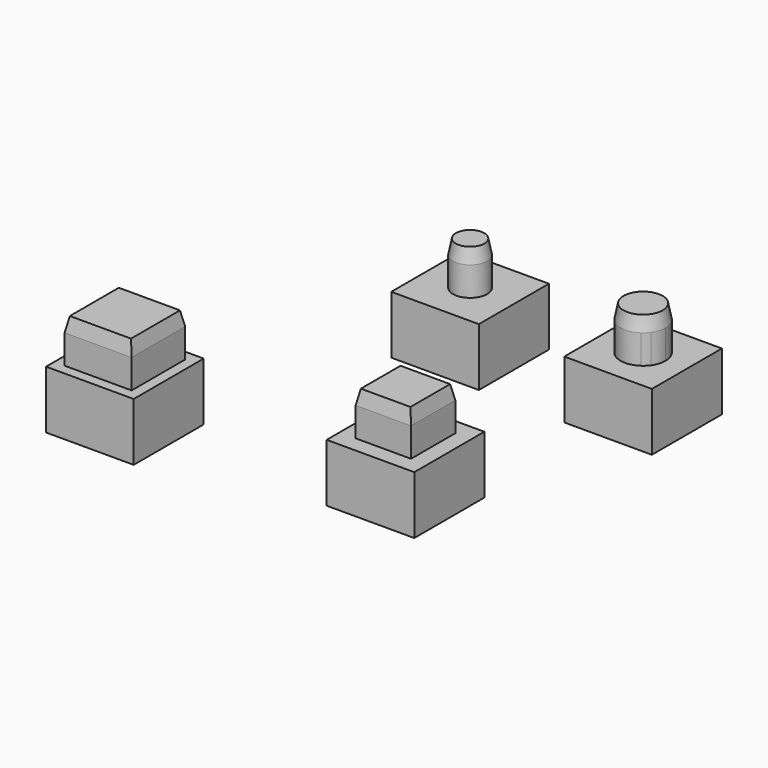
from build123d import *

# Parameters (mm, degrees)
F0_W          = 7.6708
F0_H          = 7.6708
F0_W_2        = 5.8674
F0_H_2        = 5.8674
F0_W_3        = 3.2258
F0_H_3        = 3.2258
F1_DEPTH      = 5.08
F0_R          = 1.4986
F0_W_4        = 4.8514
F0_H_4        = 4.8514
F2_DEPTH      = 8.89
F3_DEPTH      = 8.89
F4_DEPTH      = 8.89
F5_DEPTH      = 8.89
F6_C1_SIZE2   = 0.254
F6_C1_SIZE    = 1.27
F6_C2_SIZE2   = 0.254
F6_C2_SIZE    = 1.27
F6_C3_SIZE2   = 0.254
F6_C3_SIZE    = 1.27
F6_C4_SIZE2   = 0.254
F6_C4_SIZE    = 1.27
F6_4_C1_SIZE2 = 0.254
F6_4_C1_SIZE  = 1.27
F6_4_C2_SIZE2 = 0.254
F6_4_C2_SIZE  = 1.27
F6_4_C3_SIZE2 = 0.254
F6_4_C3_SIZE  = 1.27
F6_4_C4_SIZE2 = 0.254
F6_4_C4_SIZE  = 1.27
F7_DEPTH      = 3.302
F8_DEPTH      = 3.302
F9_DEPTH      = 3.302
F10_DEPTH     = 3.302


# Not quite as in the source:
# - a fillet or chamfer that OpenCascade refuses, or shapes differently, is made with other operations: its cross-section is extruded or revolved along the edge and cut away or added


with BuildPart() as f1:
    # F0 (on Top) → F1 (new body)
    with BuildSketch(Plane.XY):
        with Locations((3.9261005717, 4.6390335905)):
            Rectangle(F0_W, F0_H)
        with Locations((3.9261005717, 4.6390335905)):
            Rectangle(F0_W_2, F0_H_2, mode=Mode.SUBTRACT)
        with Locations((3.9261005717, 4.6390335905)):
            Rectangle(F0_W_2, F0_H_2)
        with Locations((3.9261005717, 4.6390335905)):
            Rectangle(F0_W_3, F0_H_3, mode=Mode.SUBTRACT)
        with Locations((3.9261005717, 4.6390335905)):
            Rectangle(F0_W_3, F0_H_3)
    extrude(amount=F1_DEPTH)

    # F0 (on Top) → F5 (join)
    with BuildSketch(Plane.XY):
        with Locations((3.9261005717, 4.6390335905)):
            Rectangle(F0_W_2, F0_H_2)
        with Locations((3.9261005717, 4.6390335905)):
            Rectangle(F0_W_3, F0_H_3, mode=Mode.SUBTRACT)
        with Locations((3.9261005717, 4.6390335905)):
            Rectangle(F0_W_3, F0_H_3)
    extrude(amount=F5_DEPTH)

    # F6: chamfer of 0.254 x 1.27 on 4 edges, made by hand

    # F6_c1
    f6_c1_edges = [f1.edges().sort_by_distance(p)[0] for p in [
        (3.9261005717, 1.7053335905, 8.89),
    ]]
    f6_c1_side = f1.faces().sort_by_distance((3.9261005717, 1.7053335905, 8.88492))[0]
    chamfer(f6_c1_edges, length=F6_C1_SIZE, length2=F6_C1_SIZE2, reference=f6_c1_side)

    # F6_c2
    f6_c2_edges = [f1.edges().sort_by_distance(p)[0] for p in [
        (6.8598005717, 4.7660335905, 8.89),
    ]]
    f6_c2_side = f1.faces().sort_by_distance((6.8598005717, 4.7660335905, 8.88492))[0]
    chamfer(f6_c2_edges, length=F6_C2_SIZE, length2=F6_C2_SIZE2, reference=f6_c2_side)

    # F6_c3
    f6_c3_edges = [f1.edges().sort_by_distance(p)[0] for p in [
        (3.7991005717, 7.5727335905, 8.89),
    ]]
    f6_c3_side = f1.faces().sort_by_distance((3.7991005717, 7.5727335905, 8.88492))[0]
    chamfer(f6_c3_edges, length=F6_C3_SIZE, length2=F6_C3_SIZE2, reference=f6_c3_side)

    # F6_c4
    f6_c4_edges = [f1.edges().sort_by_distance(p)[0] for p in [
        (0.9924005717, 4.6390335905, 8.89),
    ]]
    f6_c4_side = f1.faces().sort_by_distance((0.9924005717, 4.6390335905, 8.88492))[0]
    chamfer(f6_c4_edges, length=F6_C4_SIZE, length2=F6_C4_SIZE2, reference=f6_c4_side)

    # F0 (on Top) → F10 (cut)
    with BuildSketch(Plane.XY):
        with Locations((3.9261005717, 4.6390335905)):
            Rectangle(F0_W_3, F0_H_3)
    extrude(amount=F10_DEPTH, mode=Mode.SUBTRACT)


with BuildPart() as f1b:
    # F0 (on Top) → F1, piece 2 (new body)
    with BuildSketch(Plane.XY):
        with Locations((30.6640900671, 27.9408358037)):
            Rectangle(F0_W, F0_H)
        with BuildLine():
            Line((29.0511900671, 29.0693506862), (29.0511900671, 29.5537358037))
            Line((29.0511900671, 29.5537358037), (29.5355751847, 29.5537358037))
            ThreePointArc((29.5355751847, 29.5537358037), (30.6640900671, 29.9093358037), (31.7926049496, 29.5537358037))
            Line((31.7926049496, 29.5537358037), (32.2769900671, 29.5537358037))
            Line((32.2769900671, 29.5537358037), (32.2769900671, 29.0693506862))
            ThreePointArc((32.2769900671, 29.0693506862), (32.5415865252, 28.5324431904), (32.6325900671, 27.9408358037))
            ThreePointArc((32.6325900671, 27.9408358037), (32.5415865252, 27.349228417), (32.2769900671, 26.8123209213))
            Line((32.2769900671, 26.8123209213), (32.2769900671, 26.3279358037))
            Line((32.2769900671, 26.3279358037), (31.7926049496, 26.3279358037))
            ThreePointArc((31.7926049496, 26.3279358037), (30.6640900671, 25.9723358037), (29.5355751847, 26.3279358037))
            Line((29.5355751847, 26.3279358037), (29.0511900671, 26.3279358037))
            Line((29.0511900671, 26.3279358037), (29.0511900671, 26.8123209213))
            ThreePointArc((29.0511900671, 26.8123209213), (28.6955900671, 27.9408358037), (29.0511900671, 29.0693506862))
        make_face(mode=Mode.SUBTRACT)
        with BuildLine():
            Line((31.7926049496, 29.5537358037), (29.5355751847, 29.5537358037))
            ThreePointArc((29.5355751847, 29.5537358037), (29.2721503684, 29.3327755025), (29.0511900671, 29.0693506862))
            Line((29.0511900671, 29.0693506862), (29.0511900671, 26.8123209213))
            ThreePointArc((29.0511900671, 26.8123209213), (29.2721503684, 26.548896105), (29.5355751847, 26.3279358037))
            Line((29.5355751847, 26.3279358037), (31.7926049496, 26.3279358037))
            ThreePointArc((31.7926049496, 26.3279358037), (32.0560297659, 26.548896105), (32.2769900671, 26.8123209213))
            Line((32.2769900671, 26.8123209213), (32.2769900671, 29.0693506862))
            ThreePointArc((32.2769900671, 29.0693506862), (32.0560297659, 29.3327755025), (31.7926049496, 29.5537358037))
        make_face()
        with BuildLine():
            Line((29.0511900671, 26.8123209213), (29.0511900671, 29.0693506862))
            ThreePointArc((29.0511900671, 29.0693506862), (28.6955900671, 27.9408358037), (29.0511900671, 26.8123209213))
        make_face()
        with BuildLine():
            ThreePointArc((32.6325900671, 27.9408358037), (32.5415865252, 28.5324431904), (32.2769900671, 29.0693506862))
            Line((32.2769900671, 29.0693506862), (32.2769900671, 26.8123209213))
            ThreePointArc((32.2769900671, 26.8123209213), (32.5415865252, 27.349228417), (32.6325900671, 27.9408358037))
        make_face()
        with BuildLine():
            Line((31.7926049496, 26.3279358037), (29.5355751847, 26.3279358037))
            ThreePointArc((29.5355751847, 26.3279358037), (30.6640900671, 25.9723358037), (31.7926049496, 26.3279358037))
        make_face()
        with BuildLine():
            ThreePointArc((31.7926049496, 29.5537358037), (30.6640900671, 29.9093358037), (29.5355751847, 29.5537358037))
            Line((29.5355751847, 29.5537358037), (31.7926049496, 29.5537358037))
        make_face()
        with BuildLine():
            ThreePointArc((29.5355751847, 26.3279358037), (29.2721503684, 26.548896105), (29.0511900671, 26.8123209213))
            Line((29.0511900671, 26.8123209213), (29.0511900671, 26.3279358037))
            Line((29.0511900671, 26.3279358037), (29.5355751847, 26.3279358037))
        make_face()
        with BuildLine():
            Line((29.5355751847, 29.5537358037), (29.0511900671, 29.5537358037))
            Line((29.0511900671, 29.5537358037), (29.0511900671, 29.0693506862))
            ThreePointArc((29.0511900671, 29.0693506862), (29.2721503684, 29.3327755025), (29.5355751847, 29.5537358037))
        make_face()
        with BuildLine():
            Line((32.2769900671, 29.5537358037), (31.7926049496, 29.5537358037))
            ThreePointArc((31.7926049496, 29.5537358037), (32.0560297659, 29.3327755025), (32.2769900671, 29.0693506862))
            Line((32.2769900671, 29.0693506862), (32.2769900671, 29.5537358037))
        make_face()
        with BuildLine():
            Line((32.2769900671, 26.3279358037), (32.2769900671, 26.8123209213))
            ThreePointArc((32.2769900671, 26.8123209213), (32.0560297659, 26.548896105), (31.7926049496, 26.3279358037))
            Line((31.7926049496, 26.3279358037), (32.2769900671, 26.3279358037))
        make_face()
    extrude(amount=F1_DEPTH)

    # F0 (on Top) → F2 (join)
    with BuildSketch(Plane.XY):
        with BuildLine():
            Line((31.7926049496, 26.3279358037), (29.5355751847, 26.3279358037))
            ThreePointArc((29.5355751847, 26.3279358037), (30.6640900671, 25.9723358037), (31.7926049496, 26.3279358037))
        make_face()
        with BuildLine():
            Line((31.7926049496, 29.5537358037), (29.5355751847, 29.5537358037))
            ThreePointArc((29.5355751847, 29.5537358037), (29.2721503684, 29.3327755025), (29.0511900671, 29.0693506862))
            Line((29.0511900671, 29.0693506862), (29.0511900671, 26.8123209213))
            ThreePointArc((29.0511900671, 26.8123209213), (29.2721503684, 26.548896105), (29.5355751847, 26.3279358037))
            Line((29.5355751847, 26.3279358037), (31.7926049496, 26.3279358037))
            ThreePointArc((31.7926049496, 26.3279358037), (32.0560297659, 26.548896105), (32.2769900671, 26.8123209213))
            Line((32.2769900671, 26.8123209213), (32.2769900671, 29.0693506862))
            ThreePointArc((32.2769900671, 29.0693506862), (32.0560297659, 29.3327755025), (31.7926049496, 29.5537358037))
        make_face()
        with BuildLine():
            Line((29.0511900671, 26.8123209213), (29.0511900671, 29.0693506862))
            ThreePointArc((29.0511900671, 29.0693506862), (28.6955900671, 27.9408358037), (29.0511900671, 26.8123209213))
        make_face()
        with BuildLine():
            ThreePointArc((31.7926049496, 29.5537358037), (30.6640900671, 29.9093358037), (29.5355751847, 29.5537358037))
            Line((29.5355751847, 29.5537358037), (31.7926049496, 29.5537358037))
        make_face()
        with BuildLine():
            ThreePointArc((32.6325900671, 27.9408358037), (32.5415865252, 28.5324431904), (32.2769900671, 29.0693506862))
            Line((32.2769900671, 29.0693506862), (32.2769900671, 26.8123209213))
            ThreePointArc((32.2769900671, 26.8123209213), (32.5415865252, 27.349228417), (32.6325900671, 27.9408358037))
        make_face()
    extrude(amount=F2_DEPTH)

    # F6#2: chamfer of 0.254 x 1.27 on 1 edges, made by hand

    # F6_2_s1 → F6_2_t2 (revolve, cut)
    with BuildSketch(Plane(origin=(23.202503455, 33.1615633992, 0), x_dir=(0, 0, 1), z_dir=(-0.5732867069, -0.8193548387, 0))):
        Polygon((7.62, -11.0751608258), (8.89, -10.8211608258), (8.89, -11.0751608258), align=None)
    revolve(axis=Axis((30.6640900671, 27.9408358037, 8.89), (0, 0, 1)), mode=Mode.SUBTRACT)

    # F0 (on Top) → F7 (cut)
    with BuildSketch(Plane.XY):
        with BuildLine():
            Line((31.7926049496, 29.5537358037), (29.5355751847, 29.5537358037))
            ThreePointArc((29.5355751847, 29.5537358037), (29.2721503684, 29.3327755025), (29.0511900671, 29.0693506862))
            Line((29.0511900671, 29.0693506862), (29.0511900671, 26.8123209213))
            ThreePointArc((29.0511900671, 26.8123209213), (29.2721503684, 26.548896105), (29.5355751847, 26.3279358037))
            Line((29.5355751847, 26.3279358037), (31.7926049496, 26.3279358037))
            ThreePointArc((31.7926049496, 26.3279358037), (32.0560297659, 26.548896105), (32.2769900671, 26.8123209213))
            Line((32.2769900671, 26.8123209213), (32.2769900671, 29.0693506862))
            ThreePointArc((32.2769900671, 29.0693506862), (32.0560297659, 29.3327755025), (31.7926049496, 29.5537358037))
        make_face()
        with BuildLine():
            ThreePointArc((29.5355751847, 26.3279358037), (29.2721503684, 26.548896105), (29.0511900671, 26.8123209213))
            Line((29.0511900671, 26.8123209213), (29.0511900671, 26.3279358037))
            Line((29.0511900671, 26.3279358037), (29.5355751847, 26.3279358037))
        make_face()
        with BuildLine():
            Line((32.2769900671, 26.3279358037), (32.2769900671, 26.8123209213))
            ThreePointArc((32.2769900671, 26.8123209213), (32.0560297659, 26.548896105), (31.7926049496, 26.3279358037))
            Line((31.7926049496, 26.3279358037), (32.2769900671, 26.3279358037))
        make_face()
        with BuildLine():
            Line((32.2769900671, 29.5537358037), (31.7926049496, 29.5537358037))
            ThreePointArc((31.7926049496, 29.5537358037), (32.0560297659, 29.3327755025), (32.2769900671, 29.0693506862))
            Line((32.2769900671, 29.0693506862), (32.2769900671, 29.5537358037))
        make_face()
        with BuildLine():
            Line((29.5355751847, 29.5537358037), (29.0511900671, 29.5537358037))
            Line((29.0511900671, 29.5537358037), (29.0511900671, 29.0693506862))
            ThreePointArc((29.0511900671, 29.0693506862), (29.2721503684, 29.3327755025), (29.5355751847, 29.5537358037))
        make_face()
    extrude(amount=F7_DEPTH, mode=Mode.SUBTRACT)


with BuildPart() as f1c:
    # F0 (on Top) → F1, piece 3 (new body)
    with BuildSketch(Plane.XY):
        with Locations((15.4350250959, 28.039496392)):
            Rectangle(F0_W, F0_H)
        with Locations((15.4350250959, 28.039496392)):
            Rectangle(F0_W_3, F0_H_3, mode=Mode.SUBTRACT)
        with Locations((15.4350250959, 28.039496392)):
            Rectangle(F0_W_3, F0_H_3)
        with Locations((15.4350250959, 28.039496392)):
            Circle(F0_R, mode=Mode.SUBTRACT)
        with Locations((15.4350250959, 28.039496392)):
            Circle(F0_R)
    extrude(amount=F1_DEPTH)

    # F0 (on Top) → F3 (join)
    with BuildSketch(Plane.XY):
        with Locations((15.4350250959, 28.039496392)):
            Circle(F0_R)
    extrude(amount=F3_DEPTH)

    # F6#3: chamfer of 0.254 x 1.27 on 1 edges, made by hand

    # F6_3_s1 → F6_3_t2 (revolve, cut)
    with BuildSketch(Plane.XZ.offset(-28.039496392)):
        Polygon((16.9336250959, 7.62), (16.6796250959, 8.89), (16.9336250959, 8.89), align=None)
    revolve(axis=Axis((15.4350250959, 28.039496392, 8.89), (0, 0, 1)), mode=Mode.SUBTRACT)

    # F0 (on Top) → F8 (cut)
    with BuildSketch(Plane.XY):
        with Locations((15.4350250959, 28.039496392)):
            Rectangle(F0_W_3, F0_H_3)
        with Locations((15.4350250959, 28.039496392)):
            Circle(F0_R, mode=Mode.SUBTRACT)
        with Locations((15.4350250959, 28.039496392)):
            Circle(F0_R)
    extrude(amount=F8_DEPTH, mode=Mode.SUBTRACT)


with BuildPart() as f1d:
    # F0 (on Top) → F1, piece 4 (new body)
    with BuildSketch(Plane.XY):
        with Locations((25.6800069869, 8.162417023)):
            Rectangle(F0_W, F0_H)
        with Locations((25.6800069869, 8.162417023)):
            Rectangle(F0_W_4, F0_H_4, mode=Mode.SUBTRACT)
        with Locations((25.6800069869, 8.162417023)):
            Rectangle(F0_W_4, F0_H_4)
        with Locations((25.6800069869, 8.162417023)):
            Rectangle(F0_W_3, F0_H_3, mode=Mode.SUBTRACT)
        with Locations((25.6800069869, 8.162417023)):
            Rectangle(F0_W_3, F0_H_3)
    extrude(amount=F1_DEPTH)

    # F0 (on Top) → F4 (join)
    with BuildSketch(Plane.XY):
        with Locations((25.6800069869, 8.162417023)):
            Rectangle(F0_W_4, F0_H_4)
        with Locations((25.6800069869, 8.162417023)):
            Rectangle(F0_W_3, F0_H_3, mode=Mode.SUBTRACT)
        with Locations((25.6800069869, 8.162417023)):
            Rectangle(F0_W_3, F0_H_3)
    extrude(amount=F4_DEPTH)

    # F6#4: chamfer of 0.254 x 1.27 on 4 edges, made by hand

    # F6_4_c1
    f6_4_c1_edges = [f1d.edges().sort_by_distance(p)[0] for p in [
        (25.6800069869, 10.588117023, 8.89),
    ]]
    f6_4_c1_side = f1d.faces().sort_by_distance((25.6800069869, 10.588117023, 8.88492))[0]
    chamfer(f6_4_c1_edges, length=F6_4_C1_SIZE, length2=F6_4_C1_SIZE2, reference=f6_4_c1_side)

    # F6_4_c2
    f6_4_c2_edges = [f1d.edges().sort_by_distance(p)[0] for p in [
        (23.2543069869, 8.035417023, 8.89),
    ]]
    f6_4_c2_side = f1d.faces().sort_by_distance((23.2543069869, 8.035417023, 8.88492))[0]
    chamfer(f6_4_c2_edges, length=F6_4_C2_SIZE, length2=F6_4_C2_SIZE2, reference=f6_4_c2_side)

    # F6_4_c3
    f6_4_c3_edges = [f1d.edges().sort_by_distance(p)[0] for p in [
        (25.8070069869, 5.736717023, 8.89),
    ]]
    f6_4_c3_side = f1d.faces().sort_by_distance((25.8070069869, 5.736717023, 8.88492))[0]
    chamfer(f6_4_c3_edges, length=F6_4_C3_SIZE, length2=F6_4_C3_SIZE2, reference=f6_4_c3_side)

    # F6_4_c4
    f6_4_c4_edges = [f1d.edges().sort_by_distance(p)[0] for p in [
        (28.1057069869, 8.162417023, 8.89),
    ]]
    f6_4_c4_side = f1d.faces().sort_by_distance((28.1057069869, 8.162417023, 8.88492))[0]
    chamfer(f6_4_c4_edges, length=F6_4_C4_SIZE, length2=F6_4_C4_SIZE2, reference=f6_4_c4_side)

    # F0 (on Top) → F9 (cut)
    with BuildSketch(Plane.XY):
        with Locations((25.6800069869, 8.162417023)):
            Rectangle(F0_W_3, F0_H_3)
    extrude(amount=F9_DEPTH, mode=Mode.SUBTRACT)


solid = Compound([f1.part, f1b.part, f1c.part, f1d.part])
